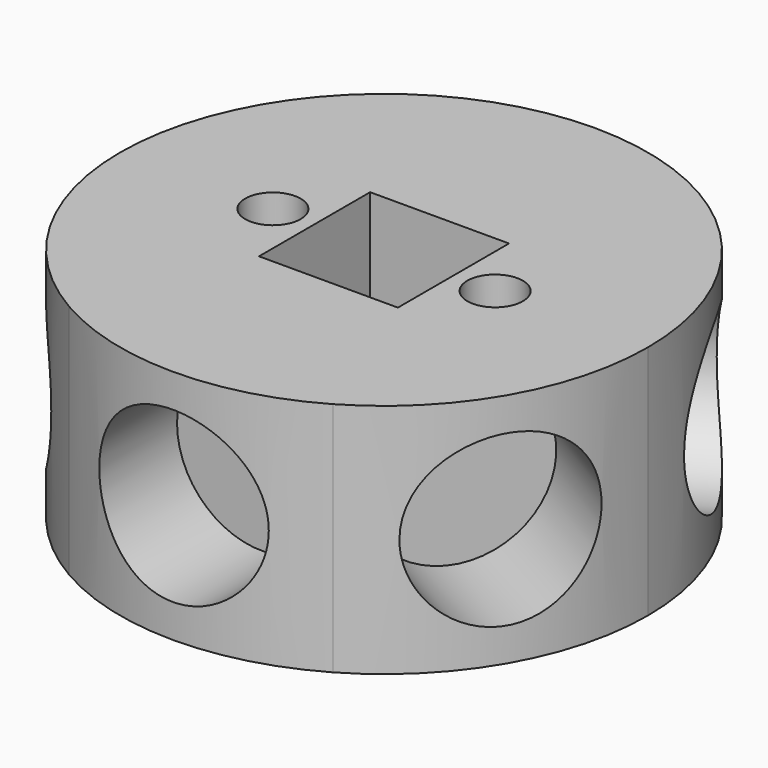
from build123d import *

# Parameters (mm, degrees)
F1_DEPTH  = 17
F5_R      = 6.1
F6_DEPTH  = 9
F7_COUNT  = 6
F9_D      = 4
F10_R     = 2
F11_DEPTH = 10
F12_DEPTH = 17.0010001


with BuildPart() as f1:
    # F0 (on Top) → F1 (new body)
    with BuildSketch(Plane.XY):
        with BuildLine():
            Line((0, 0), (9.5, 16.4544826719))
            ThreePointArc((9.5, 16.4544826719), (0, 19), (-9.5, 16.4544826719))
            Line((-9.5, 16.4544826719), (0, 0))
        make_face()
    extrude(amount=F1_DEPTH)

    # F5 (on offset) → F6 (cut)
    with BuildSketch(Plane.XZ.offset(-20)):
        with Locations((0, 8.5)):
            Circle(F5_R)
    extrude(amount=F6_DEPTH, mode=Mode.SUBTRACT)

    # F7: F1 ×6 about axis
    f7_axis = Axis((0, 0, 0), (0, 0, 1))


with BuildPart() as f1_1:
    add(f1.part)
    for i in range(1, F7_COUNT):
        add(f1.part.rotate(f7_axis, i * 360 / F7_COUNT))

    # F9 (through all)
    with Locations(Plane(origin=(0, 0, 0), x_dir=(1, 0, 0), z_dir=(0, 0, -1))):
        with Locations((-8, 0), (8, 0)):
            Hole(F9_D / 2)

    # F10 (on face) → F11 (cut)
    with BuildSketch(Plane(origin=(0, 0, 0), x_dir=(1, 0, 0), z_dir=(0, 0, -1))):
        Polygon((-5, -1.7320508076), (-5, 1.7320508076), (-8, 3.4641016151), (-11, 1.7320508076), (-11, -1.7320508076), (-8, -3.4641016151), align=None)
        with Locations((-8, 0)):
            Circle(F10_R, mode=Mode.SUBTRACT)
        Polygon((5, 1.7320508076), (5, -1.7320508076), (8, -3.4641016151), (11, -1.7320508076), (11, 1.7320508076), (8, 3.4641016151), align=None)
        with Locations((8, 0)):
            Circle(F10_R, mode=Mode.SUBTRACT)
    extrude(amount=-F11_DEPTH, mode=Mode.SUBTRACT)

    # F8 (on face) → F12 (cut, through all)
    with BuildSketch(Plane(origin=(0, 0, 0), x_dir=(1, 0, 0), z_dir=(0, 0, -1))):
        with BuildLine():
            Line((0, 2.1), (0, 5))
            Line((0, 5), (-5, 5))
            Line((-5, 5), (-5, -5))
            Line((-5, -5), (5, -5))
            Line((5, -5), (5, 5))
            Line((5, 5), (2.8867513459, 5))
            Line((2.8867513459, 5), (1.05, 1.8186533479))
            ThreePointArc((1.05, 1.8186533479), (1.0751032483, 1.8039271065), (1.1, 1.788854382))
            ThreePointArc((1.1, 1.788854382), (1.833030278, 1.0246950766), (2.1, 0))
            ThreePointArc((2.1, 0), (1.833030278, -1.0246950766), (1.1, -1.788854382))
            ThreePointArc((1.1, -1.788854382), (0, -2.1), (-1.1, -1.788854382))
            ThreePointArc((-1.1, -1.788854382), (-2.1, 0), (-1.1, 1.788854382))
            ThreePointArc((-1.1, 1.788854382), (-0.5715793024, 2.020716977), (0, 2.1))
        make_face()
        with BuildLine():
            Line((2.8867513459, 5), (0, 5))
            Line((0, 5), (0, 2.1))
            ThreePointArc((0, 2.1), (0.5435199947, 2.0284442352), (1.05, 1.8186533479))
            Line((1.05, 1.8186533479), (2.8867513459, 5))
        make_face()
        with BuildLine():
            Line((0, 0), (0, 2.1))
            ThreePointArc((0, 2.1), (-0.5715793024, 2.020716977), (-1.1, 1.788854382))
            Line((-1.1, 1.788854382), (-1.1, -1.788854382))
            ThreePointArc((-1.1, -1.788854382), (0, -2.1), (1.1, -1.788854382))
            Line((1.1, -1.788854382), (1.1, 1.788854382))
            ThreePointArc((1.1, 1.788854382), (1.0751032483, 1.8039271065), (1.05, 1.8186533479))
            Line((1.05, 1.8186533479), (0, 0))
        make_face()
        with BuildLine():
            Line((-1.1, -1.788854382), (-1.1, 1.788854382))
            ThreePointArc((-1.1, 1.788854382), (-2.1, 0), (-1.1, -1.788854382))
        make_face()
        with BuildLine():
            ThreePointArc((2.1, 0), (1.833030278, 1.0246950766), (1.1, 1.788854382))
            Line((1.1, 1.788854382), (1.1, -1.788854382))
            ThreePointArc((1.1, -1.788854382), (1.833030278, -1.0246950766), (2.1, 0))
        make_face()
        with BuildLine():
            ThreePointArc((1.05, 1.8186533479), (0.5435199947, 2.0284442352), (0, 2.1))
            Line((0, 2.1), (0, 0))
            Line((0, 0), (1.05, 1.8186533479))
        make_face()
    extrude(amount=-F12_DEPTH, mode=Mode.SUBTRACT)


solid = f1_1.part
